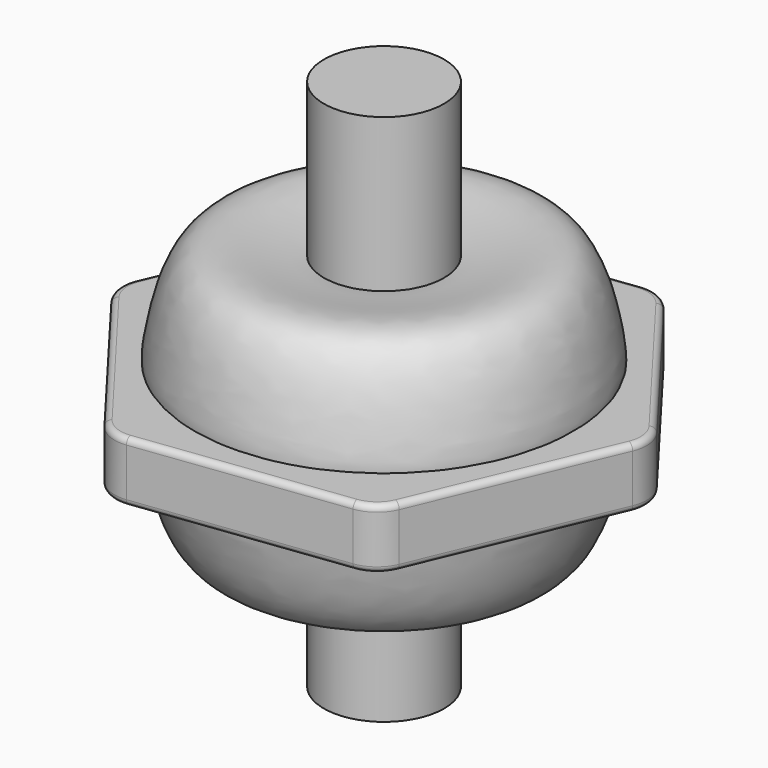
from build123d import *

# Parameters (mm, degrees)
F8_DEPTH  = 25
F9_R      = 30
F10_R     = 5
F12_R     = 50
F13_DEPTH = 443


# Not quite as in the source:
# - a feature names something its author has since deleted; it is built from what else it names
# - the program builds the solid bodies; features that only make, move or delete a surface that nothing else refers to are left out


with BuildPart() as f4:
    # F3 (on Front) → F4 (revolve)
    with BuildSketch(Plane.XZ):
        with BuildLine():
            add(Edge.make_bspline(
                [(-26.6096331179, -134.3492567539), (-18.2784247962, -120.8804854669), (-29.9815447108, -73.3605660468), (-21.7123194688, -27.679959609), (-74.7236870412, -26.6532322909), (-137.4430886255, -8.554998099), (-156.3585418602, -84.452004453), (-161.5144273247, -129.8181314401), (-79.5519521234, -149.485301482), (-34.3380070388, -146.8434468812), (-26.6096331179, -134.3492567539)],
                knots=[0, 0, 0, 0, 0.1344458877, 0.2402377282, 0.3534852575, 0.4811732516, 0.6196441183, 0.7253768662, 0.8752824258, 1, 1, 1, 1], degree=3))
        make_face()
    revolve(axis=Axis((0, 0, -51.9318208098), (0, 0, -1)))


with BuildPart() as f6_1:
    # F6: instance of F4
    add(f4.part.mirror(Plane.XY.offset(-130)))


with BuildPart() as f8:
    # F7 (on offset) → F8 (new body, symmetric)
    with BuildSketch(Plane.XY.offset(-130)):
        Polygon((125.2586688438, -165.1139688894), (205.6222259998, 25.9202048182), (80.363557156, 191.0341737077), (-125.2586688438, 165.1139688894), (-205.6222259998, -25.9202048182), (-80.363557156, -191.0341737077), align=None)
    extrude(amount=F8_DEPTH, both=True)

    # F9
    f9_edges = [f8.edges().sort_by_distance(p)[0] for p in [
        (125.258669, -165.113969, -130),
        (-80.363557, -191.034174, -130),
        (-205.622226, -25.920205, -130),
        (-125.258669, 165.113969, -130),
        (80.363557, 191.034174, -130),
        (205.622226, 25.920205, -130),
    ]]
    fillet(f9_edges, radius=F9_R)

    # F10
    f10_edges = [f8.edges().sort_by_distance(p)[0] for p in [
        (22.447556, -178.074071, -155),
        (-78.563946, -186.756274, -155),
        (-142.992892, -108.477189, -155),
        (-201.01765, -25.339764, -155),
        (-165.440447, 69.596882, -155),
        (-122.453704, 161.41651, -155),
        (122.453704, -161.41651, -155),
        (-22.447556, 178.074071, -155),
        (165.440447, -69.596882, -155),
        (78.563946, 186.756274, -155),
        (201.01765, 25.339764, -155),
        (142.992892, 108.477189, -155),
        (-142.992892, -108.477189, -105),
        (-201.01765, -25.339764, -105),
        (-78.563946, -186.756274, -105),
        (-165.440447, 69.596882, -105),
        (22.447556, -178.074071, -105),
        (-122.453704, 161.41651, -105),
        (122.453704, -161.41651, -105),
        (-22.447556, 178.074071, -105),
        (165.440447, -69.596882, -105),
        (78.563946, 186.756274, -105),
        (201.01765, 25.339764, -105),
        (142.992892, 108.477189, -105),
    ]]
    fillet(f10_edges, radius=F10_R)


with BuildPart() as f13:
    # F12 (on offset) → F13 (new body)
    with BuildSketch(Plane.XY.offset(100)):
        Circle(F12_R)
    extrude(amount=-F13_DEPTH)


solid = Compound([f4.part, f6_1.part, f8.part, f13.part])
